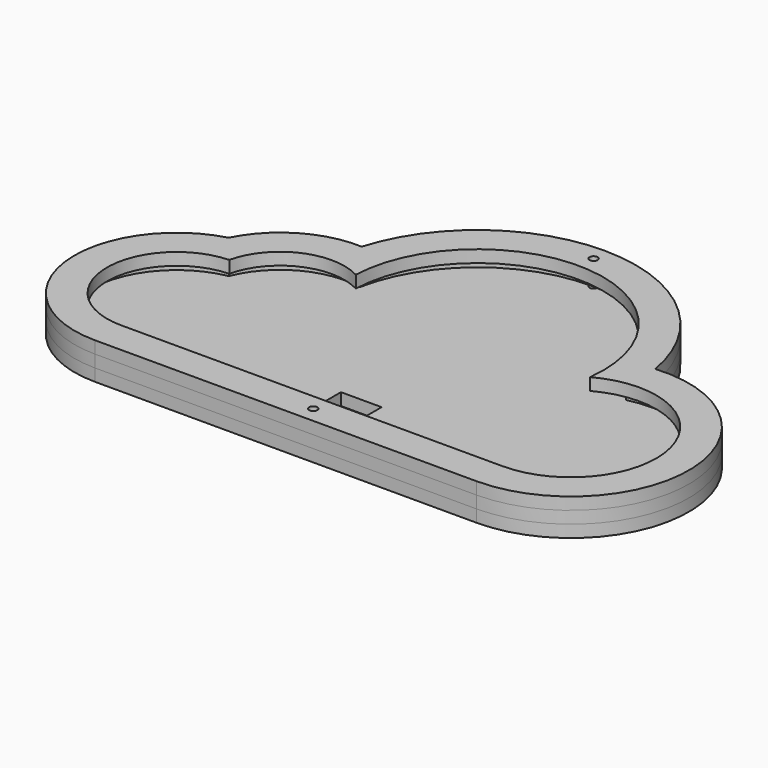
from build123d import *

# Parameters (mm, degrees)
F1_W     = 10
F1_H     = 5
F2_DEPTH = 3
F4_DEPTH = 3
F6_DEPTH = 3
F7_R     = 1
F8_DEPTH = 9.001


with BuildPart() as f2:
    # F1 (on Top) → F2 (new body)
    with BuildSketch(Plane.XY):
        with BuildLine():
            ThreePointArc((18.9239778624, 22.528357261), (-17.196872912, 54.8158089274), (-56.8917024575, 27.0396338283))
            ThreePointArc((-56.8917024575, 27.0396338283), (-69.9604581217, 23.7945983478), (-79.1795119252, 13.9797281576))
            ThreePointArc((-79.1795119252, 13.9797281576), (-97.4749227856, -13.5855716738), (-72.5783757035, -35.3738657037))
            Line((-72.5783757035, -35.3738657037), (21.3033701587, -35.3738657037))
            ThreePointArc((21.3033701587, -35.3738657037), (50.2789155891, -5.1831654845), (18.9239778624, 22.528357261))
        make_face()
        with Locations((-24.3944358081, -16.2119916081)):
            Rectangle(F1_W, F1_H, mode=Mode.SUBTRACT)
    extrude(amount=F2_DEPTH)


with BuildPart() as f4:
    # F3 (on face) → F4 (new body)
    with BuildSketch(Plane.XY.offset(3)):
        with BuildLine():
            ThreePointArc((21.3033701587, -35.3738657037), (50.2789155891, -5.1831654845), (18.9239778624, 22.528357261))
            ThreePointArc((18.9239778624, 22.528357261), (-17.196872912, 54.8158089274), (-56.8917024575, 27.0396338283))
            ThreePointArc((-56.8917024575, 27.0396338283), (-69.9604581217, 23.7945983478), (-79.1795119252, 13.9797281576))
            ThreePointArc((-79.1795119252, 13.9797281576), (-97.4749227856, -13.5855716738), (-72.5783757035, -35.3738657037))
            Line((-72.5783757035, -35.3738657037), (21.3033701587, -35.3738657037))
        make_face()
        with BuildLine():
            ThreePointArc((-76.3507281586, 10.522983545), (-67.3209277766, 20.6904762333), (-53.8633061169, 22.641789065))
            ThreePointArc((-53.8633061169, 22.641789065), (-17.1379062519, 50.8039618254), (15.4353030162, 17.9276936704))
            ThreePointArc((15.4353030162, 17.9276936704), (46.1281459316, -3.4191224282), (21.3033701587, -31.3738657037))
            Line((21.3033701587, -31.3738657037), (-72.5783757035, -31.3738657037))
            ThreePointArc((-72.5783757035, -31.3738657037), (-93.6115436771, -12.149418004), (-76.3507281586, 10.522983545))
        make_face(mode=Mode.SUBTRACT)
    extrude(amount=F4_DEPTH)


with BuildPart() as f6:
    # F5 (on face) → F6 (new body)
    with BuildSketch(Plane.XY.offset(6)):
        with BuildLine():
            ThreePointArc((18.9239778624, 22.528357261), (-17.196872912, 54.8158089274), (-56.8917024575, 27.0396338283))
            ThreePointArc((-56.8917024575, 27.0396338283), (-69.9604581217, 23.7945983478), (-79.1795119252, 13.9797281576))
            ThreePointArc((-79.1795119252, 13.9797281576), (-97.4749227856, -13.5855716738), (-72.5783757035, -35.3738657037))
            Line((-72.5783757035, -35.3738657037), (21.3033701587, -35.3738657037))
            ThreePointArc((21.3033701587, -35.3738657037), (50.2789155891, -5.1831654845), (18.9239778624, 22.528357261))
        make_face()
        with BuildLine():
            ThreePointArc((-73.3195503129, 6.846589606), (-64.4585036261, 17.6475443755), (-50.494744269, 17.2091416674))
            ThreePointArc((-50.494744269, 17.2091416674), (-16.9420148184, 46.7778414524), (11.2610857029, 12.0693586052))
            ThreePointArc((11.2610857029, 12.0693586052), (41.6541405432, -1.1925391596), (21.3033701587, -27.3738657037))
            Line((21.3033701587, -27.3738657037), (-72.5783757035, -27.3738657037))
            ThreePointArc((-72.5783757035, -27.3738657037), (-89.6926161293, -10.6262857825), (-73.3195503129, 6.846589606))
        make_face(mode=Mode.SUBTRACT)
    extrude(amount=F6_DEPTH)


with BuildPart() as f8_tool:
    # F7 (on face) → F8 (new body, through all)
    with BuildSketch(Plane.XY.offset(9)):
        with Locations((-22.0611357199, -31.4064599472)):
            Circle(F7_R)
        with Locations((-19.0083511606, 50.9767510554)):
            Circle(F7_R)
    extrude(amount=-F8_DEPTH)


with BuildPart() as f2_1:
    add(f2.part)

    # F8: cut by f8_tool
    add(f8_tool.part, mode=Mode.SUBTRACT)


with BuildPart() as f6_1:
    add(f6.part)

    # F8: cut by f8_tool
    add(f8_tool.part, mode=Mode.SUBTRACT)


solid = Compound([f4.part, f2_1.part, f6_1.part])
